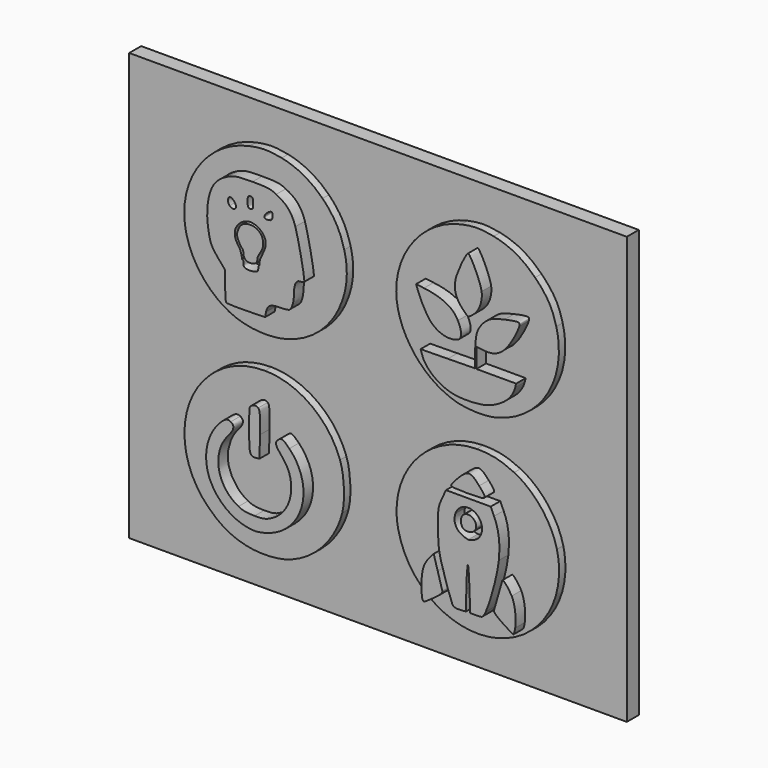
from build123d import *

# Parameters (mm, degrees)
F3_DEPTH = 4
F4_DEPTH = 1.6
F1_W     = 100
F1_H     = 85.8372836957
F5_DEPTH = 3


# Not quite as in the source:
# - ends of sketch curves that miss each other by under 0.0002 mm in the source are joined


with BuildPart() as f3:
    # F2 (on Front) → F3 (new body)
    with BuildSketch(Plane.XZ):
        with BuildLine():
            Line((10.856388, 10.649337), (11.27929, 9.450708))
            add(Edge.make_bspline(
                [(11.27929, 9.450708), (11.846181, 7.843963), (13.211307, 5.492177), (14.013125, 4.74095)],
                knots=[0, 0, 0, 0, 1, 1, 1, 1], degree=3))
            add(Edge.make_bspline(
                [(14.013125, 4.74095), (15.497278, 3.350446), (17.477149, 2.881687), (19.161384, 3.522032)],
                knots=[0, 0, 0, 0, 1, 1, 1, 1], degree=3))
            add(Edge.make_bspline(
                [(19.161384, 3.522032), (20.101494, 3.879461), (20.13529, 5.172369), (19.250312, 6.924162)],
                knots=[0, 0, 0, 0, 1, 1, 1, 1], degree=3))
            add(Edge.make_bspline(
                [(19.250312, 6.924162), (18.250619, 8.90303), (16.156947, 9.987074), (12.43714, 10.451835)],
                knots=[0, 0, 0, 0, 1, 1, 1, 1], degree=3))
            Line((12.43714, 10.451835), (10.856388, 10.649337))
        make_face()
    extrude(amount=F3_DEPTH)


with BuildPart() as f3b:
    # F2 (on Front) → F3, piece 2 (new body)
    with BuildSketch(Plane.XZ):
        with BuildLine():
            add(Edge.make_bspline(
                [(18.760442, 13.992431), (18.419317, 12.193682), (18.811394, 10.837737), (20.078044, 9.435708)],
                knots=[0, 0, 0, 0, 1, 1, 1, 1], degree=3))
            add(Edge.make_bspline(
                [(20.078044, 9.435708), (20.629055, 8.825806), (21.18236, 8.326795), (21.30761, 8.326795)],
                knots=[0, 0, 0, 0, 1, 1, 1, 1], degree=3))
            add(Edge.make_bspline(
                [(21.30761, 8.326795), (21.43286, 8.326795), (21.916956, 8.647907), (22.383382, 9.040377)],
                knots=[0, 0, 0, 0, 1, 1, 1, 1], degree=3))
            add(Edge.make_bspline(
                [(22.383382, 9.040377), (23.565721, 10.035249), (24.241581, 11.927487), (24.018569, 13.618498)],
                knots=[0, 0, 0, 0, 1, 1, 1, 1], degree=3))
            add(Edge.make_bspline(
                [(24.018569, 13.618498), (23.814508, 15.165815), (21.678117, 19.710471), (21.272612, 19.459857)],
                knots=[0, 0, 0, 0, 1, 1, 1, 1], degree=3))
            add(Edge.make_bspline(
                [(21.272612, 19.459857), (20.758084, 19.141861), (19.019372, 15.357772), (18.760442, 13.992431)],
                knots=[0, 0, 0, 0, 1, 1, 1, 1], degree=3))
        make_face()
    extrude(amount=F3_DEPTH)


with BuildPart() as f3c:
    # F2 (on Front) → F3, piece 3 (new body)
    with BuildSketch(Plane.XZ):
        with BuildLine():
            add(Edge.make_bspline(
                [(12.128999, -1.656881), (12.823372, -3.675512), (15.400976, -5.683721), (18.120153, -6.324583)],
                knots=[0, 0, 0, 0, 1, 1, 1, 1], degree=3))
            add(Edge.make_bspline(
                [(18.120153, -6.324583), (20.009315, -6.769825), (23.388692, -6.666808), (25.17971, -6.10938)],
                knots=[0, 0, 0, 0, 1, 1, 1, 1], degree=3))
            Line((25.17971, -6.10938), (25.179829, -6.10938))
            add(Edge.make_bspline(
                [(25.179829, -6.10938), (28.126489, -5.192276), (30.223222, -3.346738), (30.759464, -1.198205)],
                knots=[0, 0, 0, 0, 1, 1, 1, 1], degree=3))
            Line((30.759464, -1.198205), (30.95317, -0.422094))
            Line((30.95317, -0.422094), (26.971463, -0.422094))
            Line((26.971463, -0.422094), (22.989756, -0.422094))
            Line((22.989756, -0.422094), (22.989756, 1.540166))
            Line((22.989756, 1.540166), (22.989756, 3.502423))
            Line((22.989756, 3.502423), (24.362014, 3.3399))
            add(Edge.make_bspline(
                [(24.362014, 3.3399), (26.164198, 3.126458), (27.45279, 3.582501), (28.696676, 4.873975)],
                knots=[0, 0, 0, 0, 1, 1, 1, 1], degree=3))
            add(Edge.make_bspline(
                [(28.696676, 4.873975), (29.66311, 5.877385), (31.212408, 8.588511), (31.597173, 9.949572)],
                knots=[0, 0, 0, 0, 1, 1, 1, 1], degree=3))
            add(Edge.make_bspline(
                [(31.597173, 9.949572), (31.818026, 10.730826), (31.463515, 10.756403), (28.641677, 10.162811)],
                knots=[0, 0, 0, 0, 1, 1, 1, 1], degree=3))
            add(Edge.make_bspline(
                [(28.641677, 10.162811), (26.176398, 9.644225), (25.298966, 9.204655), (24.175936, 7.925593)],
                knots=[0, 0, 0, 0, 1, 1, 1, 1], degree=3))
            add(Edge.make_bspline(
                [(24.175936, 7.925593), (23.034243, 6.62528), (22.711022, 5.362392), (22.709109, 2.194428)],
                knots=[0, 0, 0, 0, 1, 1, 1, 1], degree=3))
            Line((22.709109, 2.194428), (22.707416, -0.410162))
            Line((22.707416, -0.410162), (17.230103, -0.486684))
            Line((17.230103, -0.486684), (11.752793, -0.563205))
            Line((11.752793, -0.563205), (12.128999, -1.656881))
        make_face()
    extrude(amount=F3_DEPTH)


with BuildPart() as f3d:
    # F2 (on Front) → F3, piece 4 (new body)
    with BuildSketch(Plane.XZ):
        with BuildLine():
            add(Edge.make_bspline(
                [(19.437499, -20.766269), (18.597241, -21.59609), (17.909756, -22.438123), (17.909756, -22.637453)],
                knots=[0, 0, 0, 0, 1, 1, 1, 1], degree=3))
            add(Edge.make_bspline(
                [(17.909756, -22.637453), (17.909756, -22.912394), (18.72719, -22.999872), (21.296423, -22.999872)],
                knots=[0, 0, 0, 0, 1, 1, 1, 1], degree=3))
            add(Edge.make_bspline(
                [(21.296423, -22.999872), (25.217988, -22.999872), (25.295182, -22.928046), (23.529489, -20.922115)],
                knots=[0, 0, 0, 0, 1, 1, 1, 1], degree=3))
            add(Edge.make_bspline(
                [(23.529489, -20.922115), (21.807547, -18.965883), (21.280841, -18.945826), (19.437499, -20.766269)],
                knots=[0, 0, 0, 0, 1, 1, 1, 1], degree=3))
        make_face()
    extrude(amount=F3_DEPTH)


with BuildPart() as f3e:
    # F2 (on Front) → F3, piece 5 (new body)
    with BuildSketch(Plane.XZ):
        with BuildLine():
            add(Edge.make_bspline(
                [(15.856011, -36.68765), (16.696635, -39.782298), (17.915336, -43.384456), (18.271681, -43.827734)],
                knots=[0, 0, 0, 0, 1, 1, 1, 1], degree=3))
            add(Edge.make_bspline(
                [(18.271681, -43.827734), (18.45048, -44.05015), (19.020374, -44.161219), (19.719797, -44.109956)],
                knots=[0, 0, 0, 0, 1, 1, 1, 1], degree=3))
            Line((19.719797, -44.109956), (20.87309, -44.025428))
            Line((20.87309, -44.025428), (20.946693, -40.074316))
            add(Edge.make_bspline(
                [(20.946693, -40.074316), (20.987175, -37.901205), (21.114175, -35.932705), (21.228915, -35.699872)],
                knots=[0, 0, 0, 0, 1, 1, 1, 1], degree=3))
            add(Edge.make_bspline(
                [(21.228915, -35.699872), (21.343656, -35.467039), (21.501034, -37.245039), (21.578645, -39.650983)],
                knots=[0, 0, 0, 0, 1, 1, 1, 1], degree=3))
            Line((21.578645, -39.650983), (21.719756, -44.025428))
            Line((21.719756, -44.025428), (22.989756, -44.025428))
            add(Edge.make_bspline(
                [(22.989756, -44.025428), (24.217482, -44.025428), (24.279822, -43.983153), (24.862597, -42.755428)],
                knots=[0, 0, 0, 0, 1, 1, 1, 1], degree=3))
            add(Edge.make_bspline(
                [(24.862597, -42.755428), (25.793544, -40.794206), (27.177923, -35.546055), (27.483925, -32.81803)],
                knots=[0, 0, 0, 0, 1, 1, 1, 1], degree=3))
            add(Edge.make_bspline(
                [(27.483925, -32.81803), (27.811828, -29.894741), (27.501191, -27.485216), (26.518336, -25.328205)],
                knots=[0, 0, 0, 0, 1, 1, 1, 1], degree=3))
            Line((26.518336, -25.328205), (25.843206, -23.846539))
            Line((25.843206, -23.846539), (21.350579, -23.846539))
            Line((21.350579, -23.846539), (16.857951, -23.846539))
            Line((16.857951, -23.846539), (16.043297, -25.610428))
            add(Edge.make_bspline(
                [(16.043297, -25.610428), (15.280992, -27.260976), (15.229102, -27.600997), (15.235678, -30.902094)],
                knots=[0, 0, 0, 0, 1, 1, 1, 1], degree=3))
            add(Edge.make_bspline(
                [(15.235678, -30.902094), (15.241111, -33.626064), (15.382453, -34.944309), (15.856011, -36.68765)],
                knots=[0, 0, 0, 0, 1, 1, 1, 1], degree=3))
        make_face()
        with BuildLine():
            add(Edge.make_bspline(
                [(18.758173, -27.369016), (18.135952, -29.254368), (19.136616, -30.729058), (21.324865, -31.151579)],
                knots=[0, 0, 0, 0, 1, 1, 1, 1], degree=3))
            add(Edge.make_bspline(
                [(23.293687, -26.36483), (21.820318, -24.891461), (19.398905, -25.427573), (18.758173, -27.369016)],
                knots=[0, 0, 0, 0, 1, 1, 1, 1], degree=3))
            add(Edge.make_bspline(
                [(22.391773, -30.871496), (24.193708, -30.24334), (24.690388, -27.761531), (23.293687, -26.36483)],
                knots=[0, 0, 0, 0, 1, 1, 1, 1], degree=3))
            add(Edge.make_bspline(
                [(21.324865, -31.151579), (21.418117, -31.169584), (21.898228, -31.043547), (22.391773, -30.871496)],
                knots=[0, 0, 0, 0, 1, 1, 1, 1], degree=3))
        make_face(mode=Mode.SUBTRACT)
    extrude(amount=F3_DEPTH)


with BuildPart() as f3f:
    # F2 (on Front) → F3, piece 6 (new body)
    with BuildSketch(Plane.XZ):
        with BuildLine():
            add(Edge.make_bspline(
                [(22.55613, -29.220132), (23.553653, -28.117882), (22.36705, -26.409695), (20.865614, -26.786529)],
                knots=[0, 0, 0, 0, 1, 1, 1, 1], degree=3))
            add(Edge.make_bspline(
                [(20.865614, -26.786529), (19.866586, -27.03727), (19.503762, -28.538187), (20.228909, -29.420428)],
                knots=[0, 0, 0, 0, 1, 1, 1, 1], degree=3))
            add(Edge.make_bspline(
                [(20.228909, -29.420428), (20.669207, -29.956111), (21.993204, -29.842161), (22.55613, -29.220132)],
                knots=[0, 0, 0, 0, 1, 1, 1, 1], degree=3))
        make_face()
    extrude(amount=F3_DEPTH)


with BuildPart() as f3g:
    # F2 (on Front) → F3, piece 7 (new body)
    with BuildSketch(Plane.XZ):
        with BuildLine():
            add(Edge.make_bspline(
                [(13.467161, -36.987838), (12.334081, -38.298619), (11.922022, -39.735432), (11.921088, -42.378861)],
                knots=[0, 0, 0, 0, 1, 1, 1, 1], degree=3))
            add(Edge.make_bspline(
                [(11.921088, -42.378861), (11.920524, -44.241051), (12.073426, -45.013205), (12.443061, -45.013205)],
                knots=[0, 0, 0, 0, 1, 1, 1, 1], degree=3))
            add(Edge.make_bspline(
                [(12.443061, -45.013205), (12.522504, -45.013205), (13.414033, -44.423403), (14.424241, -43.702534)],
                knots=[0, 0, 0, 0, 1, 1, 1, 1], degree=3))
            add(Edge.make_bspline(
                [(14.424241, -43.702534), (15.687129, -42.801356), (16.218737, -42.250264), (16.125762, -41.938645)],
                knots=[0, 0, 0, 0, 1, 1, 1, 1], degree=3))
            add(Edge.make_bspline(
                [(16.125762, -41.938645), (16.051391, -41.689375), (15.630863, -40.232756), (15.191256, -38.701712)],
                knots=[0, 0, 0, 0, 1, 1, 1, 1], degree=3))
            Line((15.191256, -38.701712), (14.391969, -35.917993))
            Line((14.391969, -35.917993), (13.467161, -36.987838))
        make_face()
    extrude(amount=F3_DEPTH)


with BuildPart() as f3h:
    # F2 (on Front) → F3, piece 8 (new body)
    with BuildSketch(Plane.XZ):
        with BuildLine():
            add(Edge.make_bspline(
                [(26.525275, -41.935484), (26.397243, -42.26363), (26.86513, -42.741441), (28.252535, -43.699373)],
                knots=[0, 0, 0, 0, 1, 1, 1, 1], degree=3))
            add(Edge.make_bspline(
                [(28.252535, -43.699373), (29.299108, -44.421981), (30.249844, -45.013205), (30.365284, -45.013205)],
                knots=[0, 0, 0, 0, 1, 1, 1, 1], degree=3))
            add(Edge.make_bspline(
                [(30.365284, -45.013205), (30.480721, -45.013205), (30.662591, -44.430244), (30.769438, -43.717738)],
                knots=[0, 0, 0, 0, 1, 1, 1, 1], degree=3))
            add(Edge.make_bspline(
                [(30.769438, -43.717738), (31.031154, -41.972504), (30.717382, -39.554793), (30.064969, -38.28954)],
                knots=[0, 0, 0, 0, 1, 1, 1, 1], degree=3))
            add(Edge.make_bspline(
                [(30.064969, -38.28954), (29.453054, -37.10283), (28.272838, -35.761312), (28.179761, -36.146675)],
                knots=[0, 0, 0, 0, 1, 1, 1, 1], degree=3))
            add(Edge.make_bspline(
                [(28.179761, -36.146675), (27.967606, -37.025027), (26.670645, -41.562912), (26.525275, -41.935484)],
                knots=[0, 0, 0, 0, 1, 1, 1, 1], degree=3))
        make_face()
    extrude(amount=F3_DEPTH)


with BuildPart() as f3i:
    # F2 (on Front) → F3, piece 9 (new body)
    with BuildSketch(Plane.XZ):
        with BuildLine():
            add(Edge.make_bspline(
                [(-28.942446, -27.138988), (-31.388401, -29.924773), (-32.050449, -34.144463), (-30.559176, -37.443494)],
                knots=[0, 0, 0, 0, 1, 1, 1, 1], degree=3))
            add(Edge.make_bspline(
                [(-30.559176, -37.443494), (-28.909863, -41.092142), (-25.403461, -43.470638), (-21.521895, -43.573745)],
                knots=[0, 0, 0, 0, 1, 1, 1, 1], degree=3))
            add(Edge.make_bspline(
                [(-21.521895, -43.573745), (-20.934915, -43.589352), (-19.665711, -43.336317), (-18.701442, -43.011476)],
                knots=[0, 0, 0, 0, 1, 1, 1, 1], degree=3))
            add(Edge.make_bspline(
                [(-18.701442, -43.011476), (-11.608941, -40.622186), (-9.46554, -32.059423), (-14.62825, -26.739316)],
                knots=[0, 0, 0, 0, 1, 1, 1, 1], degree=3))
            add(Edge.make_bspline(
                [(-14.62825, -26.739316), (-15.898536, -25.430305), (-16.254336, -25.313171), (-16.924529, -25.983364)],
                knots=[0, 0, 0, 0, 1, 1, 1, 1], degree=3))
            add(Edge.make_bspline(
                [(-16.924529, -25.983364), (-17.581836, -26.640668), (-17.488948, -26.94868), (-16.13604, -28.597967)],
                knots=[0, 0, 0, 0, 1, 1, 1, 1], degree=3))
            add(Edge.make_bspline(
                [(-16.13604, -28.597967), (-14.747283, -30.290962), (-14.263577, -31.594583), (-14.263577, -33.644391)],
                knots=[0, 0, 0, 0, 1, 1, 1, 1], degree=3))
            add(Edge.make_bspline(
                [(-14.263577, -33.644391), (-14.263577, -36.392129), (-15.66822, -38.805713), (-18.028681, -40.11394)],
                knots=[0, 0, 0, 0, 1, 1, 1, 1], degree=3))
            add(Edge.make_bspline(
                [(-18.028681, -40.11394), (-19.272505, -40.803299), (-19.793149, -40.91995), (-21.601355, -40.914399)],
                knots=[0, 0, 0, 0, 1, 1, 1, 1], degree=3))
            add(Edge.make_bspline(
                [(-21.601355, -40.914399), (-23.215008, -40.909432), (-23.986296, -40.764429), (-24.84691, -40.304172)],
                knots=[0, 0, 0, 0, 1, 1, 1, 1], degree=3))
            add(Edge.make_bspline(
                [(-24.84691, -40.304172), (-29.256997, -37.945667), (-30.253063, -32.303912), (-26.936024, -28.471368)],
                knots=[0, 0, 0, 0, 1, 1, 1, 1], degree=3))
            add(Edge.make_bspline(
                [(-26.936024, -28.471368), (-25.711732, -27.056811), (-25.55325, -26.274796), (-26.399133, -25.822094)],
                knots=[0, 0, 0, 0, 1, 1, 1, 1], degree=3))
            add(Edge.make_bspline(
                [(-26.399133, -25.822094), (-27.11782, -25.437465), (-27.724135, -25.751409), (-28.942446, -27.138988)],
                knots=[0, 0, 0, 0, 1, 1, 1, 1], degree=3))
        make_face()
    extrude(amount=F3_DEPTH)


with BuildPart() as f3j:
    # F2 (on Front) → F3, piece 10 (new body)
    with BuildSketch(Plane.XZ):
        with BuildLine():
            add(Edge.make_bspline(
                [(-22.730244, -25.90071), (-22.730244, -30.25239), (-22.591904, -30.709952), (-21.321114, -30.561446)],
                knots=[0, 0, 0, 0, 1, 1, 1, 1], degree=3))
            Line((-21.321114, -30.561446), (-20.613577, -30.478761))
            Line((-20.613577, -30.478761), (-20.53589, -26.215348))
            add(Edge.make_bspline(
                [(-20.53589, -26.215348), (-20.470699, -22.637882), (-20.528806, -21.893341), (-20.897024, -21.587745)],
                knots=[0, 0, 0, 0, 1, 1, 1, 1], degree=3))
            add(Edge.make_bspline(
                [(-20.897024, -21.587745), (-21.233882, -21.308176), (-21.49785, -21.297366), (-22.033045, -21.541218)],
                knots=[0, 0, 0, 0, 1, 1, 1, 1], degree=3))
            add(Edge.make_bspline(
                [(-22.033045, -21.541218), (-22.727252, -21.857518), (-22.730244, -21.876221), (-22.730244, -25.90071)],
                knots=[0, 0, 0, 0, 1, 1, 1, 1], degree=3))
        make_face()
    extrude(amount=F3_DEPTH)


with BuildPart() as f3k:
    # F2 (on Front) → F3, piece 11 (new body)
    with BuildSketch(Plane.XZ):
        with BuildLine():
            add(Edge.make_bspline(
                [(-24.170158, 5.663481), (-23.999101, 5.55776), (-23.859141, 5.186655), (-23.859141, 4.838805)],
                knots=[0, 0, 0, 0, 1, 1, 1, 1], degree=3))
            add(Edge.make_bspline(
                [(-23.859141, 4.838805), (-23.859141, 4.002431), (-23.349103, 3.529017), (-22.44803, 3.529017)],
                knots=[0, 0, 0, 0, 1, 1, 1, 1], degree=3))
            add(Edge.make_bspline(
                [(-22.44803, 3.529017), (-22.044452, 3.529017), (-21.561852, 3.681417), (-21.375585, 3.867684)],
                knots=[0, 0, 0, 0, 1, 1, 1, 1], degree=3))
            add(Edge.make_bspline(
                [(-21.375585, 3.867684), (-21.189254, 4.05395), (-21.036854, 4.440092), (-21.036854, 4.725777)],
                knots=[0, 0, 0, 0, 1, 1, 1, 1], degree=3))
            add(Edge.make_bspline(
                [(-21.036854, 4.725777), (-21.036854, 5.011463), (-20.790338, 5.589313), (-20.489044, 6.009889)],
                knots=[0, 0, 0, 0, 1, 1, 1, 1], degree=3))
            add(Edge.make_bspline(
                [(-20.489044, 6.009889), (-19.119718, 7.921391), (-20.161178, 10.30235), (-22.366674, 10.30235)],
                knots=[0, 0, 0, 0, 1, 1, 1, 1], degree=3))
            add(Edge.make_bspline(
                [(-22.366674, 10.30235), (-23.697809, 10.30235), (-24.401067, 9.860715), (-24.874591, 8.727412)],
                knots=[0, 0, 0, 0, 1, 1, 1, 1], degree=3))
            add(Edge.make_bspline(
                [(-24.874591, 8.727412), (-25.222438, 7.894896), (-25.223113, 7.631416), (-24.879501, 6.809026)],
                knots=[0, 0, 0, 0, 1, 1, 1, 1], degree=3))
            add(Edge.make_bspline(
                [(-24.879501, 6.809026), (-24.660424, 6.284697), (-24.341219, 5.769201), (-24.170158, 5.663481)],
                knots=[0, 0, 0, 0, 1, 1, 1, 1], degree=3))
        make_face()
    extrude(amount=F3_DEPTH)


with BuildPart() as f3l:
    # F2 (on Front) → F3, piece 12 (new body)
    with BuildSketch(Plane.XZ):
        with BuildLine():
            add(Edge.make_bspline(
                [(-12.452774, 3.529017), (-12.070036, 3.529017), (-11.69781, 3.624608), (-11.625601, 3.741446)],
                knots=[0, 0, 0, 0, 1, 1, 1, 1], degree=3))
            add(Edge.make_bspline(
                [(-11.625601, 3.741446), (-11.439698, 4.042244), (-12.729459, 10.634879), (-13.419515, 12.911063)],
                knots=[0, 0, 0, 0, 1, 1, 1, 1], degree=3))
            add(Edge.make_bspline(
                [(-13.419515, 12.911063), (-14.084239, 15.103695), (-15.153582, 16.348149), (-17.266901, 17.38849)],
                knots=[0, 0, 0, 0, 1, 1, 1, 1], degree=3))
            add(Edge.make_bspline(
                [(-17.266901, 17.38849), (-18.482478, 17.986892), (-19.022213, 18.063337), (-22.024688, 18.062366)],
                knots=[0, 0, 0, 0, 1, 1, 1, 1], degree=3))
            add(Edge.make_bspline(
                [(-22.024688, 18.062366), (-24.957942, 18.06152), (-25.604745, 17.973892), (-26.855842, 17.408607)],
                knots=[0, 0, 0, 0, 1, 1, 1, 1], degree=3))
            add(Edge.make_bspline(
                [(-26.855842, 17.408607), (-29.587231, 16.174477), (-30.748544, 14.305382), (-31.094108, 10.587248)],
                knots=[0, 0, 0, 0, 1, 1, 1, 1], degree=3))
            add(Edge.make_bspline(
                [(-31.094108, 10.587248), (-31.285554, 8.527362), (-30.844316, 5.321769), (-30.197045, 4.070085)],
                knots=[0, 0, 0, 0, 1, 1, 1, 1], degree=3))
            add(Edge.make_bspline(
                [(-30.197045, 4.070085), (-29.975311, 3.641299), (-29.28407, 2.701423), (-28.660957, 1.981471)],
                knots=[0, 0, 0, 0, 1, 1, 1, 1], degree=3))
            Line((-28.660957, 1.981471), (-27.528021, 0.672465))
            Line((-27.528021, 0.672465), (-27.528021, -2.085554))
            add(Edge.make_bspline(
                [(-27.528021, -2.085554), (-27.528021, -3.602468), (-27.439931, -4.931667), (-27.332264, -5.039332)],
                knots=[0, 0, 0, 0, 1, 1, 1, 1], degree=3))
            add(Edge.make_bspline(
                [(-27.332264, -5.039332), (-27.224599, -5.146999), (-25.419892, -5.199916), (-23.321807, -5.156925)],
                knots=[0, 0, 0, 0, 1, 1, 1, 1], degree=3))
            Line((-23.321807, -5.156925), (-19.507105, -5.078761))
            Line((-19.507105, -5.078761), (-19.308263, -4.104772))
            add(Edge.make_bspline(
                [(-19.308263, -4.104772), (-19.040428, -2.792817), (-18.402092, -2.398463), (-16.537969, -2.393329)],
                knots=[0, 0, 0, 0, 1, 1, 1, 1], degree=3))
            add(Edge.make_bspline(
                [(-16.537969, -2.393329), (-15.675109, -2.391071), (-14.818327, -2.293117), (-14.634011, -2.175919)],
                knots=[0, 0, 0, 0, 1, 1, 1, 1], degree=3))
            add(Edge.make_bspline(
                [(-14.634011, -2.175919), (-14.112574, -1.844359), (-13.699133, -0.5071), (-13.699133, 0.847906)],
                knots=[0, 0, 0, 0, 1, 1, 1, 1], degree=3))
            add(Edge.make_bspline(
                [(-13.699133, 0.847906), (-13.699133, 2.651501), (-13.291203, 3.529017), (-12.452774, 3.529017)],
                knots=[0, 0, 0, 0, 1, 1, 1, 1], degree=3))
        make_face()
        with BuildLine():
            add(Edge.make_bspline(
                [(-24.1025108844, 3.6721017677), (-23.9816326592, 3.6090354681), (-23.6790782207, 3.4636639403), (-24.2459333308, 1.9634057086), (-20.9574365071, 2.2123120207), (-20.8519988311, 2.96805549), (-20.8758805128, 3.5872974651), (-20.6810440868, 3.6736116745)],
                knots=[0, 0, 0, 0, 0.1271381056, 0.3307248938, 0.6594774476, 0.8296368057, 1, 1, 1, 1], degree=3))
            add(Edge.make_bspline(
                [(-24.1025108844, 3.6721017677), (-24.1470727205, 4.0803057171), (-24.3538814675, 4.7873489536), (-24.5777919366, 5.5036366392), (-25.5347035496, 6.6016248411), (-25.8644960912, 9.1079662141), (-22.4123561466, 11.7871995359), (-18.6332391848, 8.8711114646), (-19.9651193079, 5.9322131189), (-20.6208497732, 4.7242550949), (-20.616991922, 4.002522919), (-20.6810440868, 3.6736116745)],
                knots=[0, 0, 0, 0, 0.0875186103, 0.1572039804, 0.2528435372, 0.3755770741, 0.5295515976, 0.6855859623, 0.8222688735, 0.9184167147, 1, 1, 1, 1], degree=3))
        make_face(mode=Mode.SUBTRACT)
        with BuildLine():
            add(Edge.make_bspline(
                [(-26.652879, 13.847722), (-27.06424, 13.593493), (-27.0488, 12.75824), (-26.62491, 12.33435)],
                knots=[0, 0, 0, 0, 1, 1, 1, 1], degree=3))
            add(Edge.make_bspline(
                [(-26.652879, 13.847722), (-26.205697, 14.124096), (-25.156641, 12.981003), (-25.363275, 12.44252)],
                knots=[0, 0, 0, 0, 1, 1, 1, 1], degree=3))
            add(Edge.make_bspline(
                [(-26.62491, 12.33435), (-26.152456, 11.861905), (-25.566811, 11.912115), (-25.363275, 12.44252)],
                knots=[0, 0, 0, 0, 1, 1, 1, 1], degree=3))
        make_face(mode=Mode.SUBTRACT)
        with BuildLine():
            add(Edge.make_bspline(
                [(-23.012466, 14.253461), (-23.012466, 13.312722), (-22.918393, 13.124572), (-22.448021, 13.124572)],
                knots=[0, 0, 0, 0, 1, 1, 1, 1], degree=3))
            add(Edge.make_bspline(
                [(-22.448021, 15.38235), (-22.918393, 15.38235), (-23.012466, 15.194201), (-23.012466, 14.253461)],
                knots=[0, 0, 0, 0, 1, 1, 1, 1], degree=3))
            add(Edge.make_bspline(
                [(-21.883577, 14.253461), (-21.883577, 15.194201), (-21.97765, 15.38235), (-22.448021, 15.38235)],
                knots=[0, 0, 0, 0, 1, 1, 1, 1], degree=3))
            add(Edge.make_bspline(
                [(-22.448021, 13.124572), (-21.97765, 13.124572), (-21.883577, 13.312722), (-21.883577, 14.253461)],
                knots=[0, 0, 0, 0, 1, 1, 1, 1], degree=3))
        make_face(mode=Mode.SUBTRACT)
        with BuildLine():
            add(Edge.make_bspline(
                [(-19.625799, 12.638752), (-19.625799, 12.3707), (-19.371952, 12.269623), (-18.849688, 12.329716)],
                knots=[0, 0, 0, 0, 1, 1, 1, 1], degree=3))
            add(Edge.make_bspline(
                [(-18.244276, 13.971239), (-18.737129, 13.971239), (-19.625799, 13.11411), (-19.625799, 12.638752)],
                knots=[0, 0, 0, 0, 1, 1, 1, 1], degree=3))
            add(Edge.make_bspline(
                [(-17.984276, 13.195128), (-17.929424, 13.671849), (-18.02972, 13.971239), (-18.244276, 13.971239)],
                knots=[0, 0, 0, 0, 1, 1, 1, 1], degree=3))
            add(Edge.make_bspline(
                [(-18.849688, 12.329716), (-18.240097, 12.399857), (-18.054417, 12.585536), (-17.984276, 13.195128)],
                knots=[0, 0, 0, 0, 1, 1, 1, 1], degree=3))
        make_face(mode=Mode.SUBTRACT)
    extrude(amount=F3_DEPTH)


with BuildPart() as f4:
    # F2 (on Front) → F4 (new body)
    with BuildSketch(Plane.XZ):
        with BuildLine():
            add(Edge.make_bspline(
                [(-32.459367, -20.502016), (-39.167278, -26.789862), (-39.37288, -37.440599), (-32.911159, -43.906403)],
                knots=[0, 0, 0, 0, 1, 1, 1, 1], degree=3))
            add(Edge.make_bspline(
                [(-32.911159, -43.906403), (-30.85447, -45.96439), (-29.241359, -47.008339), (-26.775174, -47.8774)],
                knots=[0, 0, 0, 0, 1, 1, 1, 1], degree=3))
            add(Edge.make_bspline(
                [(-26.775174, -47.8774), (-23.568263, -49.007488), (-19.234126, -48.984555), (-16.12437, -47.821048)],
                knots=[0, 0, 0, 0, 1, 1, 1, 1], degree=3))
            add(Edge.make_bspline(
                [(-16.12437, -47.821048), (-11.175326, -45.969374), (-7.229956, -41.50671), (-5.908823, -36.266106)],
                knots=[0, 0, 0, 0, 1, 1, 1, 1], degree=3))
            add(Edge.make_bspline(
                [(-5.908823, -36.266106), (-5.28836, -33.804882), (-5.498068, -29.474259), (-6.356117, -27.029221)],
                knots=[0, 0, 0, 0, 1, 1, 1, 1], degree=3))
            add(Edge.make_bspline(
                [(-6.356117, -27.029221), (-8.599769, -20.635849), (-14.77449, -16.181245), (-21.4236, -16.159141)],
                knots=[0, 0, 0, 0, 1, 1, 1, 1], degree=3))
            add(Edge.make_bspline(
                [(-21.4236, -16.159141), (-25.678859, -16.145002), (-29.354273, -17.591374), (-32.459367, -20.502016)],
                knots=[0, 0, 0, 0, 1, 1, 1, 1], degree=3))
        make_face()
        with BuildLine():
            add(Edge.make_bspline(
                [(-30.559176, -37.443494), (-28.909863, -41.092142), (-25.403461, -43.470638), (-21.521895, -43.573745)],
                knots=[0, 0, 0, 0, 1, 1, 1, 1], degree=3))
            add(Edge.make_bspline(
                [(-28.942446, -27.138988), (-31.388401, -29.924773), (-32.050449, -34.144463), (-30.559176, -37.443494)],
                knots=[0, 0, 0, 0, 1, 1, 1, 1], degree=3))
            add(Edge.make_bspline(
                [(-26.399133, -25.822094), (-27.11782, -25.437465), (-27.724135, -25.751409), (-28.942446, -27.138988)],
                knots=[0, 0, 0, 0, 1, 1, 1, 1], degree=3))
            add(Edge.make_bspline(
                [(-26.936024, -28.471368), (-25.711732, -27.056811), (-25.55325, -26.274796), (-26.399133, -25.822094)],
                knots=[0, 0, 0, 0, 1, 1, 1, 1], degree=3))
            add(Edge.make_bspline(
                [(-24.84691, -40.304172), (-29.256997, -37.945667), (-30.253063, -32.303912), (-26.936024, -28.471368)],
                knots=[0, 0, 0, 0, 1, 1, 1, 1], degree=3))
            add(Edge.make_bspline(
                [(-21.601355, -40.914399), (-23.215008, -40.909432), (-23.986296, -40.764429), (-24.84691, -40.304172)],
                knots=[0, 0, 0, 0, 1, 1, 1, 1], degree=3))
            add(Edge.make_bspline(
                [(-18.028681, -40.11394), (-19.272505, -40.803299), (-19.793149, -40.91995), (-21.601355, -40.914399)],
                knots=[0, 0, 0, 0, 1, 1, 1, 1], degree=3))
            add(Edge.make_bspline(
                [(-14.263577, -33.644391), (-14.263577, -36.392129), (-15.66822, -38.805713), (-18.028681, -40.11394)],
                knots=[0, 0, 0, 0, 1, 1, 1, 1], degree=3))
            add(Edge.make_bspline(
                [(-16.13604, -28.597967), (-14.747283, -30.290962), (-14.263577, -31.594583), (-14.263577, -33.644391)],
                knots=[0, 0, 0, 0, 1, 1, 1, 1], degree=3))
            add(Edge.make_bspline(
                [(-16.924529, -25.983364), (-17.581836, -26.640668), (-17.488948, -26.94868), (-16.13604, -28.597967)],
                knots=[0, 0, 0, 0, 1, 1, 1, 1], degree=3))
            add(Edge.make_bspline(
                [(-14.62825, -26.739316), (-15.898536, -25.430305), (-16.254336, -25.313171), (-16.924529, -25.983364)],
                knots=[0, 0, 0, 0, 1, 1, 1, 1], degree=3))
            add(Edge.make_bspline(
                [(-18.701442, -43.011476), (-11.608941, -40.622186), (-9.46554, -32.059423), (-14.62825, -26.739316)],
                knots=[0, 0, 0, 0, 1, 1, 1, 1], degree=3))
            add(Edge.make_bspline(
                [(-21.521895, -43.573745), (-20.934915, -43.589352), (-19.665711, -43.336317), (-18.701442, -43.011476)],
                knots=[0, 0, 0, 0, 1, 1, 1, 1], degree=3))
        make_face(mode=Mode.SUBTRACT)
        with BuildLine():
            Line((-20.613577, -30.478761), (-21.321114, -30.561446))
            add(Edge.make_bspline(
                [(-22.730244, -25.90071), (-22.730244, -30.25239), (-22.591904, -30.709952), (-21.321114, -30.561446)],
                knots=[0, 0, 0, 0, 1, 1, 1, 1], degree=3))
            add(Edge.make_bspline(
                [(-22.033045, -21.541218), (-22.727252, -21.857518), (-22.730244, -21.876221), (-22.730244, -25.90071)],
                knots=[0, 0, 0, 0, 1, 1, 1, 1], degree=3))
            add(Edge.make_bspline(
                [(-20.897024, -21.587745), (-21.233882, -21.308176), (-21.49785, -21.297366), (-22.033045, -21.541218)],
                knots=[0, 0, 0, 0, 1, 1, 1, 1], degree=3))
            add(Edge.make_bspline(
                [(-20.53589, -26.215348), (-20.470699, -22.637882), (-20.528806, -21.893341), (-20.897024, -21.587745)],
                knots=[0, 0, 0, 0, 1, 1, 1, 1], degree=3))
            Line((-20.53589, -26.215348), (-20.613577, -30.478761))
        make_face(mode=Mode.SUBTRACT)
    extrude(amount=F4_DEPTH)


with BuildPart() as f4b:
    # F2 (on Front) → F4, piece 2 (new body)
    with BuildSketch(Plane.XZ):
        with BuildLine():
            add(Edge.make_bspline(
                [(-24.564688, 22.577775), (-33.47511, 20.707009), (-39.307176, 11.703521), (-37.25314, 2.989464)],
                knots=[0, 0, 0, 0, 1, 1, 1, 1], degree=3))
            add(Edge.make_bspline(
                [(-37.25314, 2.989464), (-36.146199, -1.706637), (-32.858852, -5.898425), (-28.565053, -8.088957)],
                knots=[0, 0, 0, 0, 1, 1, 1, 1], degree=3))
            add(Edge.make_bspline(
                [(-28.565053, -8.088957), (-25.439464, -9.683513), (-20.927623, -10.117466), (-17.251023, -9.17715)],
                knots=[0, 0, 0, 0, 1, 1, 1, 1], degree=3))
            add(Edge.make_bspline(
                [(-17.251023, -9.17715), (-12.554487, -7.975978), (-8.800266, -4.900346), (-6.651643, -0.49364)],
                knots=[0, 0, 0, 0, 1, 1, 1, 1], degree=3))
            add(Edge.make_bspline(
                [(-6.651643, -0.49364), (-4.935949, 3.025143), (-4.552576, 6.681642), (-5.507757, 10.416365)],
                knots=[0, 0, 0, 0, 1, 1, 1, 1], degree=3))
            add(Edge.make_bspline(
                [(-5.507757, 10.416365), (-6.3025, 13.523776), (-7.585144, 15.7741), (-9.880553, 18.088178)],
                knots=[0, 0, 0, 0, 1, 1, 1, 1], degree=3))
            add(Edge.make_bspline(
                [(-9.880553, 18.088178), (-12.179377, 20.405694), (-14.944187, 21.920753), (-18.073577, 22.577775)],
                knots=[0, 0, 0, 0, 1, 1, 1, 1], degree=3))
            add(Edge.make_bspline(
                [(-18.073577, 22.577775), (-20.564538, 23.100761), (-22.073727, 23.100761), (-24.564688, 22.577775)],
                knots=[0, 0, 0, 0, 1, 1, 1, 1], degree=3))
        make_face()
        with BuildLine():
            add(Edge.make_bspline(
                [(-11.625601, 3.741446), (-11.439698, 4.042244), (-12.729459, 10.634879), (-13.419515, 12.911063)],
                knots=[0, 0, 0, 0, 1, 1, 1, 1], degree=3))
            add(Edge.make_bspline(
                [(-12.452774, 3.529017), (-12.070036, 3.529017), (-11.69781, 3.624608), (-11.625601, 3.741446)],
                knots=[0, 0, 0, 0, 1, 1, 1, 1], degree=3))
            add(Edge.make_bspline(
                [(-13.699133, 0.847906), (-13.699133, 2.651501), (-13.291203, 3.529017), (-12.452774, 3.529017)],
                knots=[0, 0, 0, 0, 1, 1, 1, 1], degree=3))
            add(Edge.make_bspline(
                [(-14.634011, -2.175919), (-14.112574, -1.844359), (-13.699133, -0.5071), (-13.699133, 0.847906)],
                knots=[0, 0, 0, 0, 1, 1, 1, 1], degree=3))
            add(Edge.make_bspline(
                [(-16.537969, -2.393329), (-15.675109, -2.391071), (-14.818327, -2.293117), (-14.634011, -2.175919)],
                knots=[0, 0, 0, 0, 1, 1, 1, 1], degree=3))
            add(Edge.make_bspline(
                [(-19.308263, -4.104772), (-19.040428, -2.792817), (-18.402092, -2.398463), (-16.537969, -2.393329)],
                knots=[0, 0, 0, 0, 1, 1, 1, 1], degree=3))
            Line((-19.308263, -4.104772), (-19.507105, -5.078761))
            Line((-19.507105, -5.078761), (-23.321807, -5.156925))
            add(Edge.make_bspline(
                [(-27.332264, -5.039332), (-27.224599, -5.146999), (-25.419892, -5.199916), (-23.321807, -5.156925)],
                knots=[0, 0, 0, 0, 1, 1, 1, 1], degree=3))
            add(Edge.make_bspline(
                [(-27.528021, -2.085554), (-27.528021, -3.602468), (-27.439931, -4.931667), (-27.332264, -5.039332)],
                knots=[0, 0, 0, 0, 1, 1, 1, 1], degree=3))
            Line((-27.528021, -2.085554), (-27.528021, 0.672465))
            Line((-27.528021, 0.672465), (-28.660957, 1.981471))
            add(Edge.make_bspline(
                [(-30.197045, 4.070085), (-29.975311, 3.641299), (-29.28407, 2.701423), (-28.660957, 1.981471)],
                knots=[0, 0, 0, 0, 1, 1, 1, 1], degree=3))
            add(Edge.make_bspline(
                [(-31.094108, 10.587248), (-31.285554, 8.527362), (-30.844316, 5.321769), (-30.197045, 4.070085)],
                knots=[0, 0, 0, 0, 1, 1, 1, 1], degree=3))
            add(Edge.make_bspline(
                [(-26.855842, 17.408607), (-29.587231, 16.174477), (-30.748544, 14.305382), (-31.094108, 10.587248)],
                knots=[0, 0, 0, 0, 1, 1, 1, 1], degree=3))
            add(Edge.make_bspline(
                [(-22.024688, 18.062366), (-24.957942, 18.06152), (-25.604745, 17.973892), (-26.855842, 17.408607)],
                knots=[0, 0, 0, 0, 1, 1, 1, 1], degree=3))
            add(Edge.make_bspline(
                [(-17.266901, 17.38849), (-18.482478, 17.986892), (-19.022213, 18.063337), (-22.024688, 18.062366)],
                knots=[0, 0, 0, 0, 1, 1, 1, 1], degree=3))
            add(Edge.make_bspline(
                [(-13.419515, 12.911063), (-14.084239, 15.103695), (-15.153582, 16.348149), (-17.266901, 17.38849)],
                knots=[0, 0, 0, 0, 1, 1, 1, 1], degree=3))
        make_face(mode=Mode.SUBTRACT)
    extrude(amount=F4_DEPTH)


with BuildPart() as f4c:
    # F2 (on Front) → F4, piece 3 (new body)
    with BuildSketch(Plane.XZ):
        with BuildLine():
            add(Edge.make_bspline(
                [(28.634201, -17.874606), (25.958647, -16.57854), (24.057372, -16.142702), (21.137636, -16.15613)],
                knots=[0, 0, 0, 0, 1, 1, 1, 1], degree=3))
            add(Edge.make_bspline(
                [(21.137636, -16.15613), (11.142451, -16.202101), (3.295358, -25.757632), (5.319891, -35.41765)],
                knots=[0, 0, 0, 0, 1, 1, 1, 1], degree=3))
            add(Edge.make_bspline(
                [(5.319891, -35.41765), (7.424896, -45.461648), (17.643835, -51.258921), (27.019909, -47.72822)],
                knots=[0, 0, 0, 0, 1, 1, 1, 1], degree=3))
            add(Edge.make_bspline(
                [(27.019909, -47.72822), (34.742571, -44.820134), (39.1145, -36.662058), (37.231412, -28.673416)],
                knots=[0, 0, 0, 0, 1, 1, 1, 1], degree=3))
            add(Edge.make_bspline(
                [(37.231412, -28.673416), (36.179894, -24.212547), (32.70338, -19.845756), (28.634201, -17.874606)],
                knots=[0, 0, 0, 0, 1, 1, 1, 1], degree=3))
        make_face()
        with BuildLine():
            add(Edge.make_bspline(
                [(11.921088, -42.378861), (11.920524, -44.241051), (12.073426, -45.013205), (12.443061, -45.013205)],
                knots=[0, 0, 0, 0, 1, 1, 1, 1], degree=3))
            add(Edge.make_bspline(
                [(13.467161, -36.987838), (12.334081, -38.298619), (11.922022, -39.735432), (11.921088, -42.378861)],
                knots=[0, 0, 0, 0, 1, 1, 1, 1], degree=3))
            Line((13.467161, -36.987838), (14.391969, -35.917993))
            Line((14.391969, -35.917993), (15.191256, -38.701712))
            add(Edge.make_bspline(
                [(16.125762, -41.938645), (16.051391, -41.689375), (15.630863, -40.232756), (15.191256, -38.701712)],
                knots=[0, 0, 0, 0, 1, 1, 1, 1], degree=3))
            add(Edge.make_bspline(
                [(14.424241, -43.702534), (15.687129, -42.801356), (16.218737, -42.250264), (16.125762, -41.938645)],
                knots=[0, 0, 0, 0, 1, 1, 1, 1], degree=3))
            add(Edge.make_bspline(
                [(12.443061, -45.013205), (12.522504, -45.013205), (13.414033, -44.423403), (14.424241, -43.702534)],
                knots=[0, 0, 0, 0, 1, 1, 1, 1], degree=3))
        make_face(mode=Mode.SUBTRACT)
        with BuildLine():
            add(Edge.make_bspline(
                [(28.252535, -43.699373), (29.299108, -44.421981), (30.249844, -45.013205), (30.365284, -45.013205)],
                knots=[0, 0, 0, 0, 1, 1, 1, 1], degree=3))
            add(Edge.make_bspline(
                [(26.525275, -41.935484), (26.397243, -42.26363), (26.86513, -42.741441), (28.252535, -43.699373)],
                knots=[0, 0, 0, 0, 1, 1, 1, 1], degree=3))
            add(Edge.make_bspline(
                [(28.179761, -36.146675), (27.967606, -37.025027), (26.670645, -41.562912), (26.525275, -41.935484)],
                knots=[0, 0, 0, 0, 1, 1, 1, 1], degree=3))
            add(Edge.make_bspline(
                [(30.064969, -38.28954), (29.453054, -37.10283), (28.272838, -35.761312), (28.179761, -36.146675)],
                knots=[0, 0, 0, 0, 1, 1, 1, 1], degree=3))
            add(Edge.make_bspline(
                [(30.769438, -43.717738), (31.031154, -41.972504), (30.717382, -39.554793), (30.064969, -38.28954)],
                knots=[0, 0, 0, 0, 1, 1, 1, 1], degree=3))
            add(Edge.make_bspline(
                [(30.365284, -45.013205), (30.480721, -45.013205), (30.662591, -44.430244), (30.769438, -43.717738)],
                knots=[0, 0, 0, 0, 1, 1, 1, 1], degree=3))
        make_face(mode=Mode.SUBTRACT)
        with BuildLine():
            add(Edge.make_bspline(
                [(18.271681, -43.827734), (18.45048, -44.05015), (19.020374, -44.161219), (19.719797, -44.109956)],
                knots=[0, 0, 0, 0, 1, 1, 1, 1], degree=3))
            add(Edge.make_bspline(
                [(15.856011, -36.68765), (16.696635, -39.782298), (17.915336, -43.384456), (18.271681, -43.827734)],
                knots=[0, 0, 0, 0, 1, 1, 1, 1], degree=3))
            add(Edge.make_bspline(
                [(15.235678, -30.902094), (15.241111, -33.626064), (15.382453, -34.944309), (15.856011, -36.68765)],
                knots=[0, 0, 0, 0, 1, 1, 1, 1], degree=3))
            add(Edge.make_bspline(
                [(16.043297, -25.610428), (15.280992, -27.260976), (15.229102, -27.600997), (15.235678, -30.902094)],
                knots=[0, 0, 0, 0, 1, 1, 1, 1], degree=3))
            Line((16.043297, -25.610428), (16.857951, -23.846539))
            Line((16.857951, -23.846539), (21.350579, -23.846539))
            Line((21.350579, -23.846539), (25.843206, -23.846539))
            Line((25.843206, -23.846539), (26.518336, -25.328205))
            add(Edge.make_bspline(
                [(27.483925, -32.81803), (27.811828, -29.894741), (27.501191, -27.485216), (26.518336, -25.328205)],
                knots=[0, 0, 0, 0, 1, 1, 1, 1], degree=3))
            add(Edge.make_bspline(
                [(24.862597, -42.755428), (25.793544, -40.794206), (27.177923, -35.546055), (27.483925, -32.81803)],
                knots=[0, 0, 0, 0, 1, 1, 1, 1], degree=3))
            add(Edge.make_bspline(
                [(22.989756, -44.025428), (24.217482, -44.025428), (24.279822, -43.983153), (24.862597, -42.755428)],
                knots=[0, 0, 0, 0, 1, 1, 1, 1], degree=3))
            Line((22.989756, -44.025428), (21.719756, -44.025428))
            Line((21.719756, -44.025428), (21.578645, -39.650983))
            add(Edge.make_bspline(
                [(21.228915, -35.699872), (21.343656, -35.467039), (21.501034, -37.245039), (21.578645, -39.650983)],
                knots=[0, 0, 0, 0, 1, 1, 1, 1], degree=3))
            add(Edge.make_bspline(
                [(20.946693, -40.074316), (20.987175, -37.901205), (21.114175, -35.932705), (21.228915, -35.699872)],
                knots=[0, 0, 0, 0, 1, 1, 1, 1], degree=3))
            Line((20.946693, -40.074316), (20.87309, -44.025428))
            Line((20.87309, -44.025428), (19.719797, -44.109956))
        make_face(mode=Mode.SUBTRACT)
        with BuildLine():
            add(Edge.make_bspline(
                [(17.909756, -22.637453), (17.909756, -22.912394), (18.72719, -22.999872), (21.296423, -22.999872)],
                knots=[0, 0, 0, 0, 1, 1, 1, 1], degree=3))
            add(Edge.make_bspline(
                [(19.437499, -20.766269), (18.597241, -21.59609), (17.909756, -22.438123), (17.909756, -22.637453)],
                knots=[0, 0, 0, 0, 1, 1, 1, 1], degree=3))
            add(Edge.make_bspline(
                [(23.529489, -20.922115), (21.807547, -18.965883), (21.280841, -18.945826), (19.437499, -20.766269)],
                knots=[0, 0, 0, 0, 1, 1, 1, 1], degree=3))
            add(Edge.make_bspline(
                [(21.296423, -22.999872), (25.217988, -22.999872), (25.295182, -22.928046), (23.529489, -20.922115)],
                knots=[0, 0, 0, 0, 1, 1, 1, 1], degree=3))
        make_face(mode=Mode.SUBTRACT)
    extrude(amount=F4_DEPTH)


with BuildPart() as f4d:
    # F2 (on Front) → F4, piece 4 (new body)
    with BuildSketch(Plane.XZ):
        with BuildLine():
            add(Edge.make_bspline(
                [(18.050867, 22.577764), (10.662024, 21.026456), (4.937336, 14.065995), (4.937336, 6.63345)],
                knots=[0, 0, 0, 0, 1, 1, 1, 1], degree=3))
            add(Edge.make_bspline(
                [(4.937336, 6.63345), (4.937336, -0.576775), (10.471657, -7.581366), (17.514961, -9.285594)],
                knots=[0, 0, 0, 0, 1, 1, 1, 1], degree=3))
            add(Edge.make_bspline(
                [(17.514961, -9.285594), (19.734597, -9.822665), (23.049548, -9.833161), (25.117684, -9.309667)],
                knots=[0, 0, 0, 0, 1, 1, 1, 1], degree=3))
            add(Edge.make_bspline(
                [(25.117684, -9.309667), (34.058701, -7.046465), (39.376262, 1.828984), (37.107034, 10.701571)],
                knots=[0, 0, 0, 0, 1, 1, 1, 1], degree=3))
            add(Edge.make_bspline(
                [(37.107034, 10.701571), (36.323232, 13.766208), (35.32418, 15.472859), (32.841381, 17.988461)],
                knots=[0, 0, 0, 0, 1, 1, 1, 1], degree=3))
            add(Edge.make_bspline(
                [(32.841381, 17.988461), (30.388937, 20.473303), (27.855691, 21.872141), (24.533882, 22.575788)],
                knots=[0, 0, 0, 0, 1, 1, 1, 1], degree=3))
            add(Edge.make_bspline(
                [(24.533882, 22.575788), (22.05533, 23.100812), (20.544284, 23.101275), (18.050867, 22.577764)],
                knots=[0, 0, 0, 0, 1, 1, 1, 1], degree=3))
        make_face()
        with BuildLine():
            add(Edge.make_bspline(
                [(18.120153, -6.324583), (20.009315, -6.769825), (23.388692, -6.666808), (25.17971, -6.10938)],
                knots=[0, 0, 0, 0, 1, 1, 1, 1], degree=3))
            add(Edge.make_bspline(
                [(12.128999, -1.656881), (12.823372, -3.675512), (15.400976, -5.683721), (18.120153, -6.324583)],
                knots=[0, 0, 0, 0, 1, 1, 1, 1], degree=3))
            Line((12.128999, -1.656881), (11.752793, -0.563205))
            Line((11.752793, -0.563205), (17.230103, -0.486684))
            Line((17.230103, -0.486684), (22.707416, -0.410162))
            Line((22.707416, -0.410162), (22.709109, 2.194428))
            add(Edge.make_bspline(
                [(24.175936, 7.925593), (23.034243, 6.62528), (22.711022, 5.362392), (22.709109, 2.194428)],
                knots=[0, 0, 0, 0, 1, 1, 1, 1], degree=3))
            add(Edge.make_bspline(
                [(28.641677, 10.162811), (26.176398, 9.644225), (25.298966, 9.204655), (24.175936, 7.925593)],
                knots=[0, 0, 0, 0, 1, 1, 1, 1], degree=3))
            add(Edge.make_bspline(
                [(31.597173, 9.949572), (31.818026, 10.730826), (31.463515, 10.756403), (28.641677, 10.162811)],
                knots=[0, 0, 0, 0, 1, 1, 1, 1], degree=3))
            add(Edge.make_bspline(
                [(28.696676, 4.873975), (29.66311, 5.877385), (31.212408, 8.588511), (31.597173, 9.949572)],
                knots=[0, 0, 0, 0, 1, 1, 1, 1], degree=3))
            add(Edge.make_bspline(
                [(24.362014, 3.3399), (26.164198, 3.126458), (27.45279, 3.582501), (28.696676, 4.873975)],
                knots=[0, 0, 0, 0, 1, 1, 1, 1], degree=3))
            Line((24.362014, 3.3399), (22.989756, 3.502423))
            Line((22.989756, 3.502423), (22.989756, 1.540166))
            Line((22.989756, 1.540166), (22.989756, -0.422094))
            Line((22.989756, -0.422094), (26.971463, -0.422094))
            Line((26.971463, -0.422094), (30.95317, -0.422094))
            Line((30.95317, -0.422094), (30.759464, -1.198205))
            add(Edge.make_bspline(
                [(25.179829, -6.10938), (28.126489, -5.192276), (30.223222, -3.346738), (30.759464, -1.198205)],
                knots=[0, 0, 0, 0, 1, 1, 1, 1], degree=3))
            Line((25.179829, -6.10938), (25.17971, -6.10938))
        make_face(mode=Mode.SUBTRACT)
        with BuildLine():
            add(Edge.make_bspline(
                [(11.27929, 9.450708), (11.846181, 7.843963), (13.211307, 5.492177), (14.013125, 4.74095)],
                knots=[0, 0, 0, 0, 1, 1, 1, 1], degree=3))
            Line((11.27929, 9.450708), (10.856388, 10.649337))
            Line((10.856388, 10.649337), (12.43714, 10.451835))
            add(Edge.make_bspline(
                [(19.250312, 6.924162), (18.250619, 8.90303), (16.156947, 9.987074), (12.43714, 10.451835)],
                knots=[0, 0, 0, 0, 1, 1, 1, 1], degree=3))
            add(Edge.make_bspline(
                [(19.161384, 3.522032), (20.101494, 3.879461), (20.13529, 5.172369), (19.250312, 6.924162)],
                knots=[0, 0, 0, 0, 1, 1, 1, 1], degree=3))
            add(Edge.make_bspline(
                [(14.013125, 4.74095), (15.497278, 3.350446), (17.477149, 2.881687), (19.161384, 3.522032)],
                knots=[0, 0, 0, 0, 1, 1, 1, 1], degree=3))
        make_face(mode=Mode.SUBTRACT)
        with BuildLine():
            add(Edge.make_bspline(
                [(20.078044, 9.435708), (20.629055, 8.825806), (21.18236, 8.326795), (21.30761, 8.326795)],
                knots=[0, 0, 0, 0, 1, 1, 1, 1], degree=3))
            add(Edge.make_bspline(
                [(18.760442, 13.992431), (18.419317, 12.193682), (18.811394, 10.837737), (20.078044, 9.435708)],
                knots=[0, 0, 0, 0, 1, 1, 1, 1], degree=3))
            add(Edge.make_bspline(
                [(21.272612, 19.459857), (20.758084, 19.141861), (19.019372, 15.357772), (18.760442, 13.992431)],
                knots=[0, 0, 0, 0, 1, 1, 1, 1], degree=3))
            add(Edge.make_bspline(
                [(24.018569, 13.618498), (23.814508, 15.165815), (21.678117, 19.710471), (21.272612, 19.459857)],
                knots=[0, 0, 0, 0, 1, 1, 1, 1], degree=3))
            add(Edge.make_bspline(
                [(22.383382, 9.040377), (23.565721, 10.035249), (24.241581, 11.927487), (24.018569, 13.618498)],
                knots=[0, 0, 0, 0, 1, 1, 1, 1], degree=3))
            add(Edge.make_bspline(
                [(21.30761, 8.326795), (21.43286, 8.326795), (21.916956, 8.647907), (22.383382, 9.040377)],
                knots=[0, 0, 0, 0, 1, 1, 1, 1], degree=3))
        make_face(mode=Mode.SUBTRACT)
    extrude(amount=F4_DEPTH)


with BuildPart() as f4e:
    # F2 (on Front) → F4, piece 5 (new body)
    with BuildSketch(Plane.XZ):
        with BuildLine():
            add(Edge.make_bspline(
                [(-26.652879, 13.847722), (-26.205697, 14.124096), (-25.156641, 12.981003), (-25.363275, 12.44252)],
                knots=[0, 0, 0, 0, 1, 1, 1, 1], degree=3))
            add(Edge.make_bspline(
                [(-26.652879, 13.847722), (-27.06424, 13.593493), (-27.0488, 12.75824), (-26.62491, 12.33435)],
                knots=[0, 0, 0, 0, 1, 1, 1, 1], degree=3))
            add(Edge.make_bspline(
                [(-26.62491, 12.33435), (-26.152456, 11.861905), (-25.566811, 11.912115), (-25.363275, 12.44252)],
                knots=[0, 0, 0, 0, 1, 1, 1, 1], degree=3))
        make_face()
    extrude(amount=F4_DEPTH)


with BuildPart() as f4f:
    # F2 (on Front) → F4, piece 6 (new body)
    with BuildSketch(Plane.XZ):
        with BuildLine():
            add(Edge.make_bspline(
                [(-22.448021, 15.38235), (-22.918393, 15.38235), (-23.012466, 15.194201), (-23.012466, 14.253461)],
                knots=[0, 0, 0, 0, 1, 1, 1, 1], degree=3))
            add(Edge.make_bspline(
                [(-23.012466, 14.253461), (-23.012466, 13.312722), (-22.918393, 13.124572), (-22.448021, 13.124572)],
                knots=[0, 0, 0, 0, 1, 1, 1, 1], degree=3))
            add(Edge.make_bspline(
                [(-22.448021, 13.124572), (-21.97765, 13.124572), (-21.883577, 13.312722), (-21.883577, 14.253461)],
                knots=[0, 0, 0, 0, 1, 1, 1, 1], degree=3))
            add(Edge.make_bspline(
                [(-21.883577, 14.253461), (-21.883577, 15.194201), (-21.97765, 15.38235), (-22.448021, 15.38235)],
                knots=[0, 0, 0, 0, 1, 1, 1, 1], degree=3))
        make_face()
    extrude(amount=F4_DEPTH)


with BuildPart() as f4g:
    # F2 (on Front) → F4, piece 7 (new body)
    with BuildSketch(Plane.XZ):
        with BuildLine():
            add(Edge.make_bspline(
                [(-18.244276, 13.971239), (-18.737129, 13.971239), (-19.625799, 13.11411), (-19.625799, 12.638752)],
                knots=[0, 0, 0, 0, 1, 1, 1, 1], degree=3))
            add(Edge.make_bspline(
                [(-19.625799, 12.638752), (-19.625799, 12.3707), (-19.371952, 12.269623), (-18.849688, 12.329716)],
                knots=[0, 0, 0, 0, 1, 1, 1, 1], degree=3))
            add(Edge.make_bspline(
                [(-18.849688, 12.329716), (-18.240097, 12.399857), (-18.054417, 12.585536), (-17.984276, 13.195128)],
                knots=[0, 0, 0, 0, 1, 1, 1, 1], degree=3))
            add(Edge.make_bspline(
                [(-17.984276, 13.195128), (-17.929424, 13.671849), (-18.02972, 13.971239), (-18.244276, 13.971239)],
                knots=[0, 0, 0, 0, 1, 1, 1, 1], degree=3))
        make_face()
    extrude(amount=F4_DEPTH)


with BuildPart() as f4h:
    # F2 (on Front) → F4, piece 8 (new body)
    with BuildSketch(Plane.XZ):
        with BuildLine():
            add(Edge.make_bspline(
                [(-24.1025108844, 3.6721017677), (-24.1470727205, 4.0803057171), (-24.3538814675, 4.7873489536), (-24.5777919366, 5.5036366392), (-25.5347035496, 6.6016248411), (-25.8644960912, 9.1079662141), (-22.4123561466, 11.7871995359), (-18.6332391848, 8.8711114646), (-19.9651193079, 5.9322131189), (-20.6208497732, 4.7242550949), (-20.616991922, 4.002522919), (-20.6810440868, 3.6736116745)],
                knots=[0, 0, 0, 0, 0.0875186103, 0.1572039804, 0.2528435372, 0.3755770741, 0.5295515976, 0.6855859623, 0.8222688735, 0.9184167147, 1, 1, 1, 1], degree=3))
            add(Edge.make_bspline(
                [(-24.1025108844, 3.6721017677), (-23.9816326592, 3.6090354681), (-23.6790782207, 3.4636639403), (-24.2459333308, 1.9634057086), (-20.9574365071, 2.2123120207), (-20.8519988311, 2.96805549), (-20.8758805128, 3.5872974651), (-20.6810440868, 3.6736116745)],
                knots=[0, 0, 0, 0, 0.1271381056, 0.3307248938, 0.6594774476, 0.8296368057, 1, 1, 1, 1], degree=3))
        make_face()
        with BuildLine():
            add(Edge.make_bspline(
                [(-23.859141, 4.838805), (-23.859141, 4.002431), (-23.349103, 3.529017), (-22.44803, 3.529017)],
                knots=[0, 0, 0, 0, 1, 1, 1, 1], degree=3))
            add(Edge.make_bspline(
                [(-24.170158, 5.663481), (-23.999101, 5.55776), (-23.859141, 5.186655), (-23.859141, 4.838805)],
                knots=[0, 0, 0, 0, 1, 1, 1, 1], degree=3))
            add(Edge.make_bspline(
                [(-24.879501, 6.809026), (-24.660424, 6.284697), (-24.341219, 5.769201), (-24.170158, 5.663481)],
                knots=[0, 0, 0, 0, 1, 1, 1, 1], degree=3))
            add(Edge.make_bspline(
                [(-24.874591, 8.727412), (-25.222438, 7.894896), (-25.223113, 7.631416), (-24.879501, 6.809026)],
                knots=[0, 0, 0, 0, 1, 1, 1, 1], degree=3))
            add(Edge.make_bspline(
                [(-22.366674, 10.30235), (-23.697809, 10.30235), (-24.401067, 9.860715), (-24.874591, 8.727412)],
                knots=[0, 0, 0, 0, 1, 1, 1, 1], degree=3))
            add(Edge.make_bspline(
                [(-20.489044, 6.009889), (-19.119718, 7.921391), (-20.161178, 10.30235), (-22.366674, 10.30235)],
                knots=[0, 0, 0, 0, 1, 1, 1, 1], degree=3))
            add(Edge.make_bspline(
                [(-21.036854, 4.725777), (-21.036854, 5.011463), (-20.790338, 5.589313), (-20.489044, 6.009889)],
                knots=[0, 0, 0, 0, 1, 1, 1, 1], degree=3))
            add(Edge.make_bspline(
                [(-21.375521, 3.867684), (-21.189254, 4.05395), (-21.036854, 4.440092), (-21.036854, 4.725777)],
                knots=[0, 0, 0, 0, 1, 1, 1, 1], degree=3))
            add(Edge.make_bspline(
                [(-22.44803, 3.529017), (-22.044452, 3.529017), (-21.561852, 3.681417), (-21.375521, 3.867684)],
                knots=[0, 0, 0, 0, 1, 1, 1, 1], degree=3))
        make_face(mode=Mode.SUBTRACT)
    extrude(amount=F4_DEPTH)


with BuildPart() as f4i:
    # F2 (on Front) → F4, piece 9 (new body)
    with BuildSketch(Plane.XZ):
        with BuildLine():
            add(Edge.make_bspline(
                [(23.293687, -26.36483), (21.820318, -24.891461), (19.398905, -25.427573), (18.758173, -27.369016)],
                knots=[0, 0, 0, 0, 1, 1, 1, 1], degree=3))
            add(Edge.make_bspline(
                [(18.758173, -27.369016), (18.135952, -29.254368), (19.136616, -30.729058), (21.324865, -31.151579)],
                knots=[0, 0, 0, 0, 1, 1, 1, 1], degree=3))
            add(Edge.make_bspline(
                [(21.324865, -31.151579), (21.418117, -31.169584), (21.898228, -31.043547), (22.391773, -30.871496)],
                knots=[0, 0, 0, 0, 1, 1, 1, 1], degree=3))
            add(Edge.make_bspline(
                [(22.391773, -30.871496), (24.193708, -30.24334), (24.690388, -27.761531), (23.293687, -26.36483)],
                knots=[0, 0, 0, 0, 1, 1, 1, 1], degree=3))
        make_face()
        with BuildLine():
            add(Edge.make_bspline(
                [(20.865614, -26.786529), (19.866586, -27.03727), (19.503762, -28.538187), (20.228909, -29.420428)],
                knots=[0, 0, 0, 0, 1, 1, 1, 1], degree=3))
            add(Edge.make_bspline(
                [(22.55613, -29.220132), (23.553653, -28.117882), (22.36705, -26.409695), (20.865614, -26.786529)],
                knots=[0, 0, 0, 0, 1, 1, 1, 1], degree=3))
            add(Edge.make_bspline(
                [(20.228909, -29.420428), (20.669207, -29.956111), (21.993204, -29.842161), (22.55613, -29.220132)],
                knots=[0, 0, 0, 0, 1, 1, 1, 1], degree=3))
        make_face(mode=Mode.SUBTRACT)
    extrude(amount=F4_DEPTH)


with BuildPart() as f5:
    # F1 (on Front) → F5 (new body)
    with BuildSketch(Plane.XZ):
        with Locations((0, -12.7908300498)):
            Rectangle(F1_W, F1_H)
    extrude(amount=-F5_DEPTH)


solid = Compound([f3.part, f3b.part, f3c.part, f3d.part, f3e.part, f3f.part, f3g.part, f3h.part, f3i.part, f3j.part, f3k.part, f3l.part, f4.part, f4b.part, f4c.part, f4d.part, f4e.part, f4f.part, f4g.part, f4h.part, f4i.part, f5.part])
